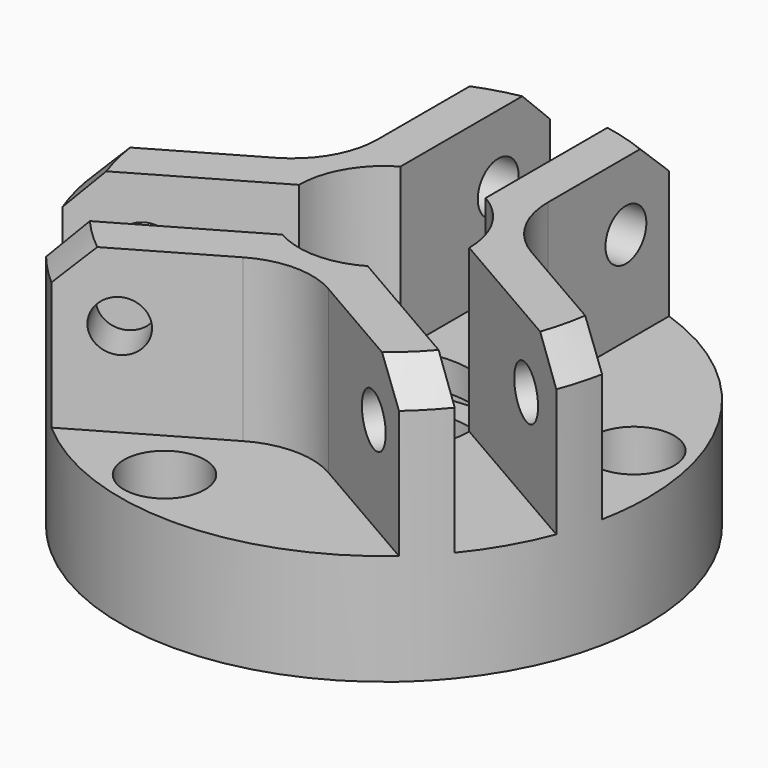
from build123d import *

# Parameters (mm, degrees)
F5_DEPTH         = 13
F6_DEPTH         = 32
F3_W             = 3
F3_H             = 2.5
F4_R             = 3
F10_DEPTH        = 12.5
F10_COPIES_COUNT = 3
F12_D            = 5.5
F12_CBORE_D      = 9.5
F12_CBORE_DEPTH  = 8


# Not quite as in the source:
# - a pattern or mirror of a feature is missing from the dataset's text; its kind, count and spacing are read off the source's solid


with BuildPart() as f5:
    # F2 (on Top) → F5 (new body, through all)
    with BuildSketch(Plane.XY):
        with BuildLine():
            Line((-10, 11.5470053838), (-10, 29.3428015022))
            ThreePointArc((-10, 29.3428015022), (-26.8467875173, 15.5), (-30.4116115191, -6.0111467133))
            Line((-30.4116115191, -6.0111467133), (-15, 2.8867513459))
            ThreePointArc((-15, 2.8867513459), (-11.3397459622, 6.5470053838), (-10, 11.5470053838))
        make_face()
    extrude(amount=F5_DEPTH)



with BuildPart() as f5b:
    # F2 (on Top) → F5, piece 2 (new body, through all)
    with BuildSketch(Plane.XY):
        with BuildLine():
            ThreePointArc((-20.4116115191, -23.331654789), (0, -31), (20.4116115191, -23.331654789))
            Line((20.4116115191, -23.331654789), (5, -14.4337567297))
            ThreePointArc((5, -14.4337567297), (0, -13.0940107676), (-5, -14.4337567297))
            Line((-5, -14.4337567297), (-20.4116115191, -23.331654789))
        make_face()
    extrude(amount=F5_DEPTH)


with BuildPart() as f5c:
    # F2 (on Top) → F5, piece 3 (new body, through all)
    with BuildSketch(Plane.XY):
        with BuildLine():
            ThreePointArc((30.4116115191, -6.0111467133), (30.852552221, -3.019937326), (31, 0))
            ThreePointArc((31, 0), (25.2091253319, 18.0416185527), (10, 29.3428015022))
            Line((10, 29.3428015022), (10, 11.5470053838))
            ThreePointArc((10, 11.5470053838), (11.3397459622, 6.5470053838), (15, 2.8867513459))
            Line((15, 2.8867513459), (30.4116115191, -6.0111467133))
        make_face()
    extrude(amount=F5_DEPTH)


with BuildPart() as f5d:
    # F2 (on Top) → F5, piece 4 (new body, through all)
    with BuildSketch(Plane.XY):
        with BuildLine():
            ThreePointArc((23.995282599, -19.6271855597), (26.8467875173, -15.5), (28.995282599, -10.9669315219))
            Line((28.995282599, -10.9669315219), (10, 0))
            ThreePointArc((10, 0), (8.6602540378, -5), (5, -8.6602540378))
            Line((5, -8.6602540378), (23.995282599, -19.6271855597))
        make_face()
    extrude(amount=F5_DEPTH)


with BuildPart() as f5e:
    # F2 (on Top) → F5, piece 5 (new body, through all)
    with BuildSketch(Plane.XY):
        with BuildLine():
            Line((5, 8.6602540378), (5, 30.5941170816))
            ThreePointArc((5, 30.5941170816), (0, 31), (-5, 30.5941170816))
            Line((-5, 30.5941170816), (-5, 8.6602540378))
            ThreePointArc((-5, 8.6602540378), (0, 10), (5, 8.6602540378))
        make_face()
    extrude(amount=F5_DEPTH)


with BuildPart() as f5f:
    # F2 (on Top) → F5, piece 6 (new body, through all)
    with BuildSketch(Plane.XY):
        with BuildLine():
            ThreePointArc((-5, -8.6602540378), (-8.6602540378, -5), (-10, 0))
            Line((-10, 0), (-28.995282599, -10.9669315219))
            ThreePointArc((-28.995282599, -10.9669315219), (-26.8467875173, -15.5), (-23.995282599, -19.6271855597))
            Line((-23.995282599, -19.6271855597), (-5, -8.6602540378))
        make_face()
    extrude(amount=F5_DEPTH)


with BuildPart() as f5_1:
    add(f5.part)

    add(f5b.part)  # F6 merges F5b

    add(f5c.part)  # F6 merges F5c

    add(f5d.part)  # F6 merges F5d

    add(f5e.part)  # F6 merges F5e

    add(f5f.part)  # F6 merges F5f
    # F2 (on Top) → F6 (join, through all)
    with BuildSketch(Plane.XY):
        with BuildLine():
            ThreePointArc((20.4116115191, -23.331654789), (22.280570782, -21.5540289883), (23.995282599, -19.6271855597))
            Line((23.995282599, -19.6271855597), (5, -8.6602540378))
            ThreePointArc((5, -8.6602540378), (0, -10), (-5, -8.6602540378))
            Line((-5, -8.6602540378), (-23.995282599, -19.6271855597))
            ThreePointArc((-23.995282599, -19.6271855597), (-22.280570782, -21.5540289883), (-20.4116115191, -23.331654789))
            Line((-20.4116115191, -23.331654789), (-5, -14.4337567297))
            ThreePointArc((-5, -14.4337567297), (0, -13.0940107676), (5, -14.4337567297))
            Line((5, -14.4337567297), (20.4116115191, -23.331654789))
        make_face()
        with BuildLine():
            Line((10, 11.5470053838), (10, 29.3428015022))
            ThreePointArc((10, 29.3428015022), (7.5260512668, 30.0725548022), (5, 30.5941170816))
            Line((5, 30.5941170816), (5, 8.6602540378))
            ThreePointArc((5, 8.6602540378), (8.6602540378, 5), (10, 0))
            Line((10, 0), (28.995282599, -10.9669315219))
            ThreePointArc((28.995282599, -10.9669315219), (29.8066220488, -8.5185258139), (30.4116115191, -6.0111467133))
            Line((30.4116115191, -6.0111467133), (15, 2.8867513459))
            ThreePointArc((15, 2.8867513459), (11.3397459622, 6.5470053838), (10, 11.5470053838))
        make_face()
        with BuildLine():
            Line((-5, 8.6602540378), (-5, 30.5941170816))
            ThreePointArc((-5, 30.5941170816), (-7.5260512668, 30.0725548022), (-10, 29.3428015022))
            Line((-10, 29.3428015022), (-10, 11.5470053838))
            ThreePointArc((-10, 11.5470053838), (-11.3397459622, 6.5470053838), (-15, 2.8867513459))
            Line((-15, 2.8867513459), (-30.4116115191, -6.0111467133))
            ThreePointArc((-30.4116115191, -6.0111467133), (-29.8066220488, -8.5185258139), (-28.995282599, -10.9669315219))
            Line((-28.995282599, -10.9669315219), (-10, 0))
            ThreePointArc((-10, 0), (-8.6602540378, 5), (-5, 8.6602540378))
        make_face()
    extrude(amount=F6_DEPTH)

    # F7: union 

    # F3 (on Front) → F8 (revolve, cut)
    with BuildSketch(Plane.XZ):
        with Locations((11.5, 8.25)):
            Rectangle(F3_W, F3_H)
    revolve(axis=Axis((0, 0, 6.5), (0, 0, 1)), mode=Mode.SUBTRACT)

    # F3 (on Front) → F9 (revolve, cut)
    with BuildSketch(Plane.XZ):
        Polygon((27, 32), (31, 28), (31, 32), align=None)
    revolve(axis=Axis((0, 0, 6.5), (0, 0, 1)), mode=Mode.SUBTRACT)

    # F4 (on Right) → F10 (cut, symmetric)
    with BuildSketch(Plane.YZ):
        with Locations((23, 24)):
            Circle(F4_R)
    f10 = extrude(amount=F10_DEPTH, both=True, mode=Mode.SUBTRACT)

    # F10_copies: F10 ×3 about axis
    f10_copies_axis = Axis((0, 0, 0), (0, 0, 1))
    for i in range(1, F10_COPIES_COUNT):
        add(f10.rotate(f10_copies_axis, i * 360 / F10_COPIES_COUNT), mode=Mode.SUBTRACT)

    # F12 (through all)
    with Locations(Plane.XY.offset(13)):
        with Locations((-6.4704761276, -24.1481456572), (24.1481456572, 6.4704761276), (-17.6776695297, 17.6776695297)):
            CounterBoreHole(F12_D / 2, F12_CBORE_D / 2, F12_CBORE_DEPTH)


solid = f5_1.part
